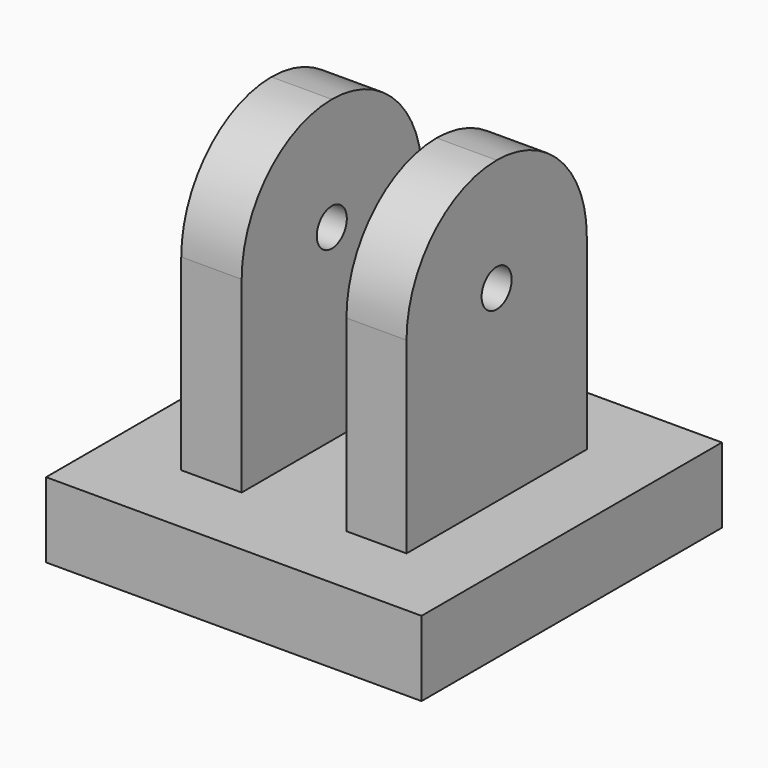
from build123d import *

# Parameters (mm, degrees)
F0_W     = 50
F0_H     = 50
F1_DEPTH = 10
F2_W     = 8.0474452116
F2_H     = 30
F2_W_2   = 8
F3_DEPTH = 40
F4_R     = 14.99999
F6_D     = 5


# Not quite as in the source:
# - a fillet or chamfer is up to 0.001 mm smaller than in the source, because OpenCascade refuses the exact size


with BuildPart() as f1:
    # F0 (on Top) → F1 (new body)
    with BuildSketch(Plane.XY):
        with Locations((2.2992696613, -1.7406867517)):
            Rectangle(F0_W, F0_H)
    extrude(amount=F1_DEPTH)

    # F2 (on face) → F3 (join)
    with BuildSketch(Plane.XY.offset(10)):
        with Locations((-8.6770077329, -1.7406867517)):
            Rectangle(F2_W, F2_H)
        with Locations((13.2992696613, -1.7406867517)):
            Rectangle(F2_W_2, F2_H)
    extrude(amount=F3_DEPTH)

    # F4 (radius 15 in the source; OpenCascade refuses exactly that, so slightly less here)
    f4_edges = [f1.edges().sort_by_distance(p)[0] for p in [
        (-8.677008, -16.740687, 50),
        (13.29927, -16.740687, 50),
        (-8.677008, 13.259313, 50),
        (13.29927, 13.259313, 50),
    ]]
    fillet(f4_edges, radius=F4_R)

    # F6 (through all)
    with Locations(Plane.YZ.offset(17.2992696613)):
        with Locations((-1.7406867517, 35)):
            Hole(F6_D / 2)


solid = f1.part
